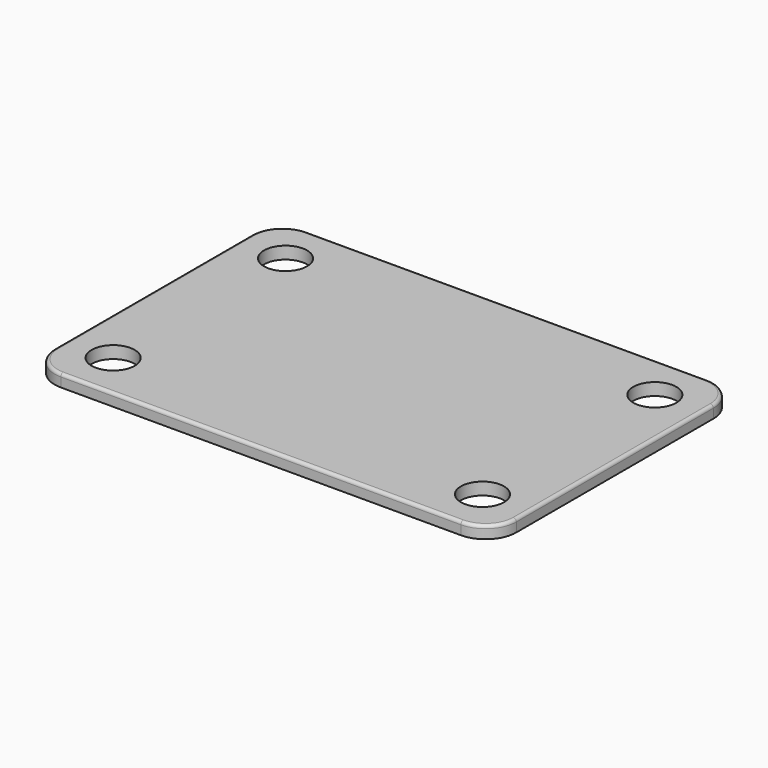
from build123d import *

# Parameters (mm, degrees)
F0_R     = 3.5
F1_DEPTH = 2
F2_R     = 0.5


with BuildPart() as f1:
    # F0 (on Top) → F1 (new body)
    with BuildSketch(Plane.XY):
        with BuildLine():
            ThreePointArc((38.0882352941, 20.5882352941), (36.6237692001, 24.1237692001), (33.0882352941, 25.5882352941))
            Line((33.0882352941, 25.5882352941), (-31.9117647059, 25.5882352941))
            ThreePointArc((-31.9117647059, 25.5882352941), (-35.4472986118, 24.1237692001), (-36.9117647059, 20.5882352941))
            Line((-36.9117647059, 20.5882352941), (-36.9117647059, -19.4117647059))
            ThreePointArc((-36.9117647059, -19.4117647059), (-35.4472986118, -22.9472986118), (-31.9117647059, -24.4117647059))
            Line((-31.9117647059, -24.4117647059), (33.0882352941, -24.4117647059))
            ThreePointArc((33.0882352941, -24.4117647059), (36.6237692001, -22.9472986118), (38.0882352941, -19.4117647059))
            Line((38.0882352941, -19.4117647059), (38.0882352941, 20.5882352941))
        make_face()
        with BuildLine():
            ThreePointArc((33.0882352941, 24.5882352941), (35.9166624189, 23.4166624189), (37.0882352941, 20.5882352941))
            Line((37.0882352941, 20.5882352941), (37.0882352941, -19.4117647059))
            ThreePointArc((37.0882352941, -19.4117647059), (35.9166624189, -22.2401918306), (33.0882352941, -23.4117647059))
            Line((33.0882352941, -23.4117647059), (-31.9117647059, -23.4117647059))
            ThreePointArc((-31.9117647059, -23.4117647059), (-34.7401918306, -22.2401918306), (-35.9117647059, -19.4117647059))
            Line((-35.9117647059, -19.4117647059), (-35.9117647059, 20.5882352941))
            ThreePointArc((-35.9117647059, 20.5882352941), (-34.7401918306, 23.4166624189), (-31.9117647059, 24.5882352941))
            Line((-31.9117647059, 24.5882352941), (33.0882352941, 24.5882352941))
        make_face(mode=Mode.SUBTRACT)
        with BuildLine():
            Line((37.0882352941, -19.4117647059), (37.0882352941, 20.5882352941))
            ThreePointArc((37.0882352941, 20.5882352941), (35.9166624189, 23.4166624189), (33.0882352941, 24.5882352941))
            Line((33.0882352941, 24.5882352941), (-31.9117647059, 24.5882352941))
            ThreePointArc((-31.9117647059, 24.5882352941), (-34.7401918306, 23.4166624189), (-35.9117647059, 20.5882352941))
            Line((-35.9117647059, 20.5882352941), (-35.9117647059, -19.4117647059))
            ThreePointArc((-35.9117647059, -19.4117647059), (-34.7401918306, -22.2401918306), (-31.9117647059, -23.4117647059))
            Line((-31.9117647059, -23.4117647059), (33.0882352941, -23.4117647059))
            ThreePointArc((33.0882352941, -23.4117647059), (35.9166624189, -22.2401918306), (37.0882352941, -19.4117647059))
        make_face()
        with BuildLine():
            ThreePointArc((33.0882352941, 23.0882352941), (34.8560022471, 22.3560022471), (35.5882352941, 20.5882352941))
            Line((35.5882352941, 20.5882352941), (35.5882352941, -19.4117647059))
            ThreePointArc((35.5882352941, -19.4117647059), (34.8560022471, -21.1795316588), (33.0882352941, -21.9117647059))
            Line((33.0882352941, -21.9117647059), (-31.9117647059, -21.9117647059))
            ThreePointArc((-31.9117647059, -21.9117647059), (-33.6795316588, -21.1795316588), (-34.4117647059, -19.4117647059))
            Line((-34.4117647059, -19.4117647059), (-34.4117647059, 20.5882352941))
            ThreePointArc((-34.4117647059, 20.5882352941), (-33.6795316588, 22.3560022471), (-31.9117647059, 23.0882352941))
            Line((-31.9117647059, 23.0882352941), (33.0882352941, 23.0882352941))
        make_face(mode=Mode.SUBTRACT)
        with BuildLine():
            Line((35.5882352941, -19.4117647059), (35.5882352941, 20.5882352941))
            ThreePointArc((35.5882352941, 20.5882352941), (34.8560022471, 22.3560022471), (33.0882352941, 23.0882352941))
            Line((33.0882352941, 23.0882352941), (-31.9117647059, 23.0882352941))
            ThreePointArc((-31.9117647059, 23.0882352941), (-33.6795316588, 22.3560022471), (-34.4117647059, 20.5882352941))
            Line((-34.4117647059, 20.5882352941), (-34.4117647059, -19.4117647059))
            ThreePointArc((-34.4117647059, -19.4117647059), (-33.6795316588, -21.1795316588), (-31.9117647059, -21.9117647059))
            Line((-31.9117647059, -21.9117647059), (33.0882352941, -21.9117647059))
            ThreePointArc((33.0882352941, -21.9117647059), (34.8560022471, -21.1795316588), (35.5882352941, -19.4117647059))
        make_face()
        with BuildLine():
            ThreePointArc((33.0882352941, 22.0882352941), (34.1488954659, 21.6488954659), (34.5882352941, 20.5882352941))
            Line((34.5882352941, 20.5882352941), (34.5882352941, 14.3133180765))
            Line((34.5882352941, 14.3133180765), (34.5882352941, -13.1368474882))
            Line((34.5882352941, -13.1368474882), (34.5882352941, -19.4117647059))
            ThreePointArc((34.5882352941, -19.4117647059), (34.1488954659, -20.4724248777), (33.0882352941, -20.9117647059))
            Line((33.0882352941, -20.9117647059), (26.8133180765, -20.9117647059))
            Line((26.8133180765, -20.9117647059), (-25.6368474882, -20.9117647059))
            Line((-25.6368474882, -20.9117647059), (-31.9117647059, -20.9117647059))
            ThreePointArc((-31.9117647059, -20.9117647059), (-32.9724248777, -20.4724248777), (-33.4117647059, -19.4117647059))
            Line((-33.4117647059, -19.4117647059), (-33.4117647059, -13.1368474882))
            Line((-33.4117647059, -13.1368474882), (-33.4117647059, 14.3133180765))
            Line((-33.4117647059, 14.3133180765), (-33.4117647059, 20.5882352941))
            ThreePointArc((-33.4117647059, 20.5882352941), (-32.9724248777, 21.6488954659), (-31.9117647059, 22.0882352941))
            Line((-31.9117647059, 22.0882352941), (-25.6368474882, 22.0882352941))
            Line((-25.6368474882, 22.0882352941), (26.8133180765, 22.0882352941))
            Line((26.8133180765, 22.0882352941), (33.0882352941, 22.0882352941))
        make_face(mode=Mode.SUBTRACT)
        with BuildLine():
            Line((34.5882352941, -13.1368474882), (34.5882352941, 14.3133180765))
            ThreePointArc((34.5882352941, 14.3133180765), (26.6991479976, 14.1991479976), (26.8133180765, 22.0882352941))
            Line((26.8133180765, 22.0882352941), (-25.6368474882, 22.0882352941))
            ThreePointArc((-25.6368474882, 22.0882352941), (-25.5226774094, 14.1991479976), (-33.4117647059, 14.3133180765))
            Line((-33.4117647059, 14.3133180765), (-33.4117647059, -13.1368474882))
            ThreePointArc((-33.4117647059, -13.1368474882), (-25.5226774094, -13.0226774094), (-25.6368474882, -20.9117647059))
            Line((-25.6368474882, -20.9117647059), (26.8133180765, -20.9117647059))
            ThreePointArc((26.8133180765, -20.9117647059), (26.6991479976, -13.0226774094), (34.5882352941, -13.1368474882))
        make_face()
        with BuildLine():
            ThreePointArc((-33.4117647059, 14.3133180765), (-25.5226774094, 14.1991479976), (-25.6368474882, 22.0882352941))
            Line((-25.6368474882, 22.0882352941), (-31.9117647059, 22.0882352941))
            ThreePointArc((-31.9117647059, 22.0882352941), (-32.9724248777, 21.6488954659), (-33.4117647059, 20.5882352941))
            Line((-33.4117647059, 20.5882352941), (-33.4117647059, 14.3133180765))
        make_face()
        with Locations((-29.4117647059, 18.0882352941)):
            Circle(F0_R, mode=Mode.SUBTRACT)
        with BuildLine():
            Line((-31.9117647059, -20.9117647059), (-25.6368474882, -20.9117647059))
            ThreePointArc((-25.6368474882, -20.9117647059), (-25.5226774094, -13.0226774094), (-33.4117647059, -13.1368474882))
            Line((-33.4117647059, -13.1368474882), (-33.4117647059, -19.4117647059))
            ThreePointArc((-33.4117647059, -19.4117647059), (-32.9724248777, -20.4724248777), (-31.9117647059, -20.9117647059))
        make_face()
        with Locations((-29.4117647059, -16.9117647059)):
            Circle(F0_R, mode=Mode.SUBTRACT)
        with BuildLine():
            Line((34.5882352941, 14.3133180765), (34.5882352941, 20.5882352941))
            ThreePointArc((34.5882352941, 20.5882352941), (34.1488954659, 21.6488954659), (33.0882352941, 22.0882352941))
            Line((33.0882352941, 22.0882352941), (26.8133180765, 22.0882352941))
            ThreePointArc((26.8133180765, 22.0882352941), (26.6991479976, 14.1991479976), (34.5882352941, 14.3133180765))
        make_face()
        with Locations((30.5882352941, 18.0882352941)):
            Circle(F0_R, mode=Mode.SUBTRACT)
        with BuildLine():
            Line((34.5882352941, -19.4117647059), (34.5882352941, -13.1368474882))
            ThreePointArc((34.5882352941, -13.1368474882), (26.6991479976, -13.0226774094), (26.8133180765, -20.9117647059))
            Line((26.8133180765, -20.9117647059), (33.0882352941, -20.9117647059))
            ThreePointArc((33.0882352941, -20.9117647059), (34.1488954659, -20.4724248777), (34.5882352941, -19.4117647059))
        make_face()
        with Locations((30.5882352941, -16.9117647059)):
            Circle(F0_R, mode=Mode.SUBTRACT)
    extrude(amount=F1_DEPTH)

    # F2
    f2_edges = [f1.edges().sort_by_distance(p)[0] for p in [
        (-36.911765, 0.588235, 2),
    ]]
    fillet(f2_edges, radius=F2_R)


solid = f1.part
